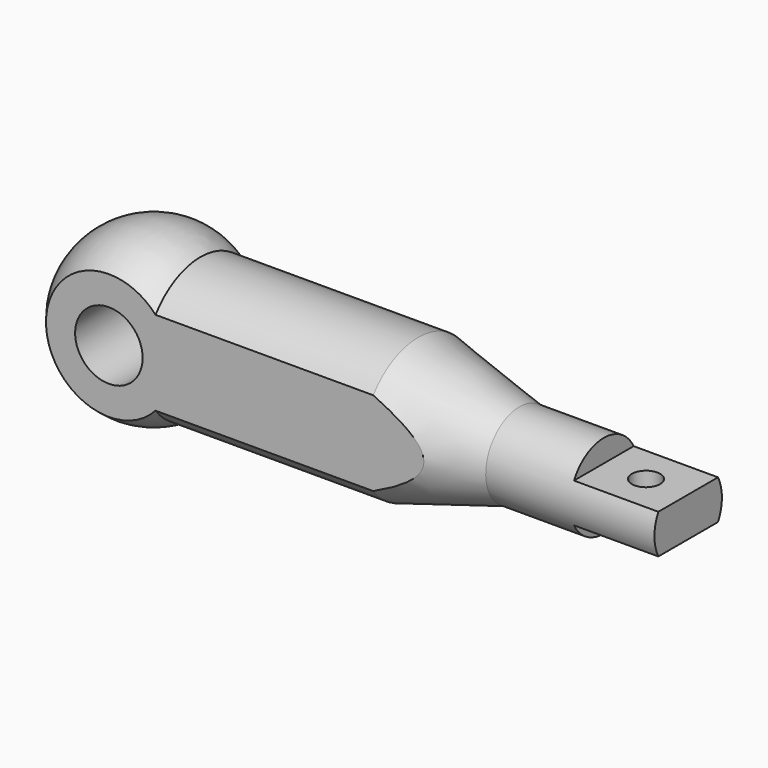
from build123d import *

# Parameters (mm, degrees)
F2_W          = 381
F2_H          = 101.6
F3_DEPTH      = 381.001
F3_DEPTH_BACK = 381.001
F5_DEPTH      = 2794.001
F6_R          = 152.4
F7_DEPTH      = 508.001
F8_R          = 63.5
F9_DEPTH      = 469.901


with BuildPart() as f1:
    # F0 (on Front) → F1 (revolve)
    with BuildSketch(Plane.XZ):
        with BuildLine():
            ThreePointArc((210.605674, 317.5), (-180.16692, 335.709519), (-381, 0))
            Line((-381, 0), (2413, 0))
            Line((2413, 0), (2413, 190.5))
            Line((2413, 190.5), (1651, 190.5))
            Line((1651, 190.5), (1193.8, 317.5))
            Line((1193.8, 317.5), (210.605674, 317.5))
        make_face()
    revolve(axis=Axis((1407.305002, 0, 0), (1, 0, 0)))

    # F2 (on Front) → F3 (cut, two sides)
    with BuildSketch(Plane.XZ) as f3_sk:
        with Locations((2222.5, 139.7)):
            Rectangle(F2_W, F2_H)
        with Locations((2222.5, -139.7)):
            Rectangle(F2_W, F2_H)
    extrude(amount=-F3_DEPTH, mode=Mode.SUBTRACT)
    extrude(f3_sk.sketch, amount=F3_DEPTH_BACK, mode=Mode.SUBTRACT)

    # F4 (on face) → F5 (cut, through all)
    with BuildSketch(Plane.YZ.offset(2413)):
        with BuildLine():
            Line((-254, -283.980633), (-254, 283.980633))
            ThreePointArc((-254, 283.980633), (-381, 0), (-254, -283.980633))
        make_face()
        with BuildLine():
            ThreePointArc((254, -283.980633), (381, 0), (254, 283.980633))
            Line((254, 283.980633), (254, -283.980633))
        make_face()
    extrude(amount=-F5_DEPTH, mode=Mode.SUBTRACT)

    # F6 (on face) → F7 (cut, through all)
    with BuildSketch(Plane.XZ.offset(254)):
        Circle(F6_R)
    extrude(amount=-F7_DEPTH, mode=Mode.SUBTRACT)

    # F8 (on face) → F9 (cut, through all)
    with BuildSketch(Plane.XY.offset(88.9)):
        with Locations((2222.5, 0)):
            Circle(F8_R)
    extrude(amount=-F9_DEPTH, mode=Mode.SUBTRACT)


solid = f1.part
